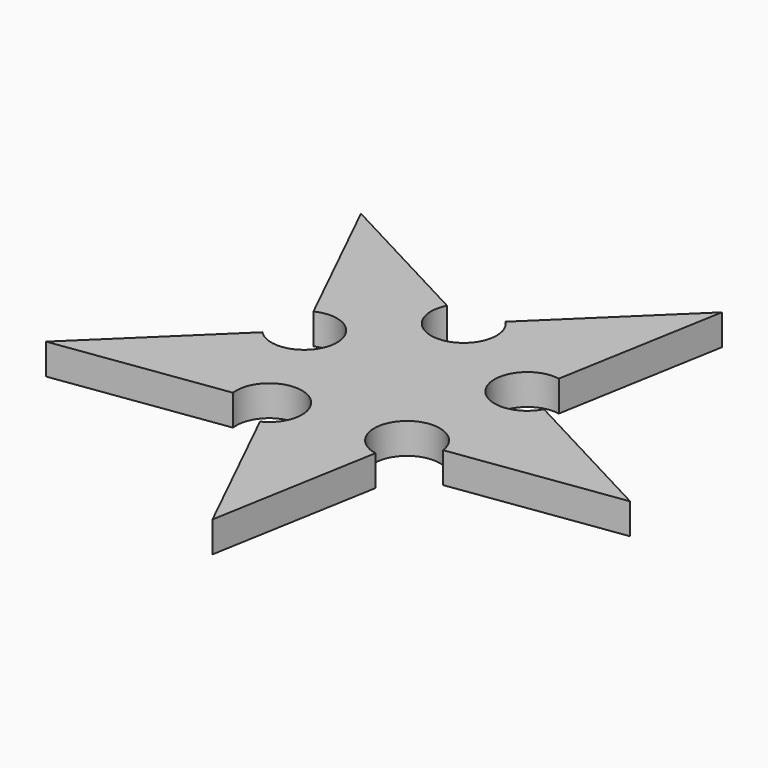
from build123d import *

# Parameters (mm, degrees)
F1_DEPTH = 4.7625


# Not quite as in the source:
# - a feature of the source that left no trace in its solid (it failed there, or was rolled back) is left out


with BuildPart() as f1:
    # F0 (on Top) → F1 (new body)
    with BuildSketch(Plane.XY):
        with BuildLine():
            Line((-6.7869197201, 18.6999163445), (-29.9817704813, 31.019788517))
            Line((-29.9817704813, 31.019788517), (-18.4581812066, 7.4192113543))
            ThreePointArc((-18.4581812066, 7.4192113543), (-11.2260431578, 1.9743769297), (-19.8819508265, -0.6761522815))
            Line((-19.8819508265, -0.6761522815), (-38.7664486034, -18.9287163727))
            Line((-38.7664486034, -18.9287163727), (-12.7599809824, -15.2621111222))
            ThreePointArc((-12.7599809824, -15.2621111222), (-5.3467821599, -10.0664854729), (-5.5008016534, -19.117801436))
            Line((-5.5008016534, -19.117801436), (6.0227876213, -42.7183785987))
            Line((6.0227876213, -42.7183785987), (10.5720792637, -16.8517147679))
            ThreePointArc((10.5720792637, -16.8517147679), (7.9215500525, -8.1958070991), (16.4822684394, -11.1392987961))
            Line((16.4822684394, -11.1392987961), (42.4887360604, -7.4726935456))
            Line((42.4887360604, -7.4726935456), (19.2938852991, 4.8471786269))
            ThreePointArc((19.2938852991, 4.8471786269), (10.242569336, 5.0011981203), (15.6874037606, 12.2333361692))
            Line((15.6874037606, 12.2333361692), (20.236695403, 38.1))
            Line((20.236695403, 38.1), (1.3521976262, 19.8474359089))
            ThreePointArc((1.3521976262, 19.8474359089), (-1.5912940708, 11.286717522), (-6.7869197201, 18.6999163445))
        make_face()
    extrude(amount=F1_DEPTH)


solid = f1.part
